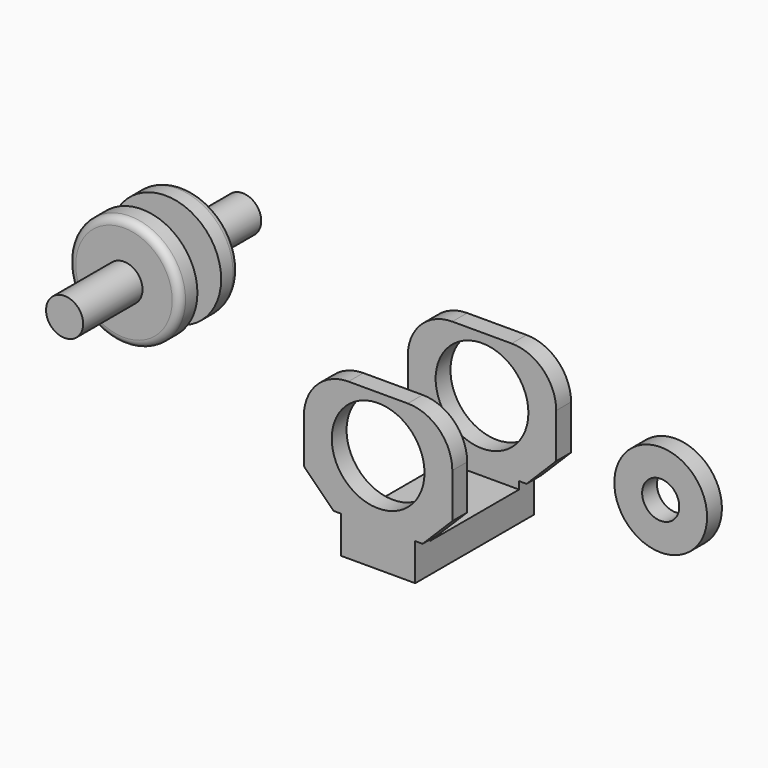
from build123d import *

# Parameters (mm, degrees)
F0_W      = 25.4
F0_H      = 25.4
F1_DEPTH  = 26.67
F2_W      = 25.4
F2_H      = 19.05
F3_DEPTH  = 21.59
F4_R      = 7.9375
F4_W      = 6.35
F4_H      = 6.35
F5_DEPTH  = 25.4
F6_R      = 7.62
F7_R      = 9.525
F7_R_2    = 3.175
F8_DEPTH  = 3.81
F9_R      = 1.27
F10_DEPTH = 16.51
F11_DEPTH = 2.54
F12_R     = 3.175
F12_R_2   = 2.286
F13_DEPTH = 0.64135
F15_SIZE  = 5.08
F16_R     = 7.9375
F16_R_2   = 3.175
F17_DEPTH = 3.175


with BuildPart() as f1:
    # F0 (on Top) → F1 (new body)
    with BuildSketch(Plane.XY):
        Rectangle(F0_W, F0_H)
    extrude(amount=F1_DEPTH)

    # F2 (on face) → F3 (cut)
    with BuildSketch(Plane.XY.offset(26.67)):
        Rectangle(F2_W, F2_H)
    extrude(amount=-F3_DEPTH, mode=Mode.SUBTRACT)

    # F4 (on face) → F5 (cut)
    with BuildSketch(Plane.XZ.offset(12.7)):
        with Locations((0, 17.145)):
            Circle(F4_R)
        with Locations((-9.525, 3.175)):
            Rectangle(F4_W, F4_H)
        with Locations((9.525, 3.175)):
            Rectangle(F4_W, F4_H)
    extrude(amount=-F5_DEPTH, mode=Mode.SUBTRACT)

    # F6
    f6_edges = [f1.edges().sort_by_distance(p)[0] for p in [
        (12.7, -11.1125, 26.67),
        (-12.7, -11.1125, 26.67),
        (12.7, 11.1125, 26.67),
        (-12.7, 11.1125, 26.67),
    ]]
    fillet(f6_edges, radius=F6_R)

    # F15
    f15_edges = [f1.edges().sort_by_distance(p)[0] for p in [
        (12.7, -11.1125, 6.35),
        (-12.7, -11.1125, 6.35),
        (-12.7, 11.1125, 6.35),
        (12.7, 11.1125, 6.35),
    ]]
    chamfer(f15_edges, length=F15_SIZE)


with BuildPart() as f8:
    # F7 (on Front) → F8 (new body)
    with BuildSketch(Plane.XZ):
        with Locations((-50.6110191345, 23.1454782188)):
            Circle(F7_R)
        with Locations((-50.6110191345, 23.1454782188)):
            Circle(F7_R_2, mode=Mode.SUBTRACT)
    extrude(amount=F8_DEPTH)

    # F9
    f9_edges = [f8.edges().sort_by_distance(p)[0] for p in [
        (-60.136019, -3.81, 23.145478),
    ]]
    fillet(f9_edges, radius=F9_R)

    # F7 (on Front) → F10 (join)
    with BuildSketch(Plane.XZ):
        with Locations((-50.6110191345, 23.1454782188)):
            Circle(F7_R_2)
    extrude(amount=F10_DEPTH)

    # F7 (on Front) → F11 (join)
    with BuildSketch(Plane.XZ):
        with Locations((-50.6110191345, 23.1454782188)):
            Circle(F7_R_2)
    extrude(amount=-F11_DEPTH)

    # F12 (on face) → F13 (cut, symmetric)
    with BuildSketch(Plane(origin=(0, 2.54, 0), x_dir=(-1, 0, 0), z_dir=(0, 1, 0))):
        with Locations((50.6110191345, 23.1454782188)):
            Circle(F12_R)
        with Locations((50.6110191345, 23.1454782188)):
            Circle(F12_R_2, mode=Mode.SUBTRACT)
    extrude(amount=F13_DEPTH, both=True, mode=Mode.SUBTRACT)

    # F14: F8 across face


with BuildPart() as f8_1:
    add(f8.part)
    add(f8.part.mirror(Plane(origin=(-50.6110191345, 2.54, 23.1454782188), x_dir=(1, 0, 0), z_dir=(0, 1, 0))))


with BuildPart() as f17:
    # F16 (on Front) → F17 (new body)
    with BuildSketch(Plane.XZ):
        with Locations((40.7415293157, 19.8798608035)):
            Circle(F16_R)
        with Locations((40.7415293157, 19.8798608035)):
            Circle(F16_R_2, mode=Mode.SUBTRACT)
    extrude(amount=F17_DEPTH)


solid = Compound([f1.part, f8_1.part, f17.part])
